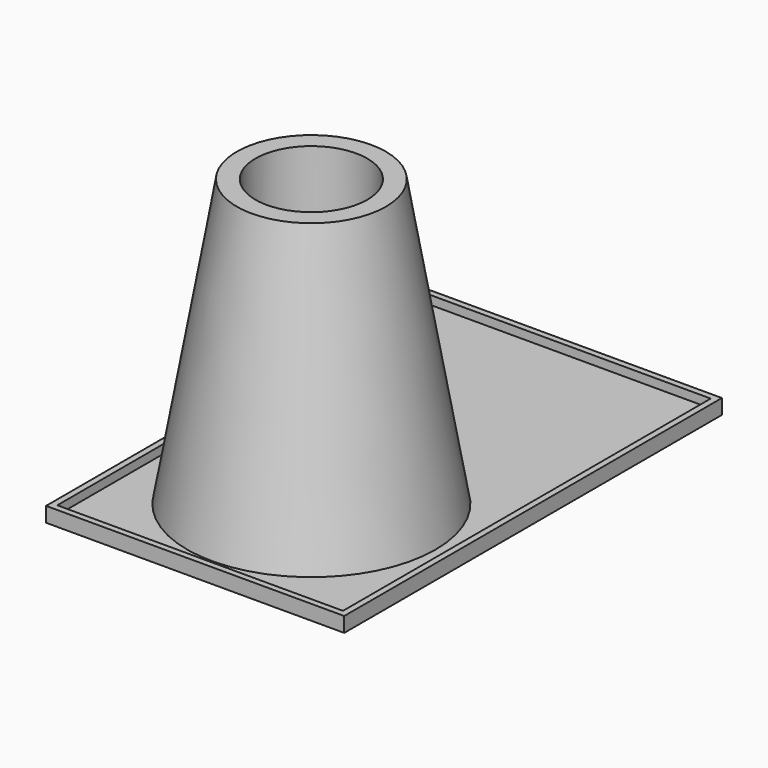
from build123d import *

# Parameters (mm, degrees)
F0_W     = 120
F0_H     = 190
F1_DEPTH = 6
F2_T     = -2.5
F3_R     = 50
F4_DEPTH = 115
F5_SIZE2 = 114.99999
F5_SIZE  = 19.99999
F6_R     = 22.5
F7_DEPTH = 25


# Not quite as in the source:
# - a fillet or chamfer is up to 0.001 mm smaller than in the source, because OpenCascade refuses the exact size


with BuildPart() as f1:
    # F0 (on Top) → F1 (new body)
    with BuildSketch(Plane.XY):
        with Locations((0, 36.5384568274)):
            Rectangle(F0_W, F0_H)
    extrude(amount=F1_DEPTH)

    # F2
    f2_openings = [f1.faces().sort_by_distance(p)[0] for p in [
        (0, 36.538457, 6),
    ]]
    offset(amount=F2_T, openings=f2_openings)

    # F3 (on face) → F4 (join)
    with BuildSketch(Plane.XY.offset(2.5)):
        Circle(F3_R)
    extrude(amount=F4_DEPTH)

    # F5 (size 20 and 115 in the source; OpenCascade refuses exactly that, so slightly less here)
    f5_edges = [f1.edges().sort_by_distance(p)[0] for p in [
        (-50, 0, 117.5),
    ]]
    f5_side = f1.faces().sort_by_distance((0, 0, 117.5))[0]
    chamfer(f5_edges, length=F5_SIZE, length2=F5_SIZE2, reference=f5_side)

    # F6 (on face) → F7 (cut)
    with BuildSketch(Plane.XY.offset(117.5)):
        Circle(F6_R)
    extrude(amount=-F7_DEPTH, mode=Mode.SUBTRACT)


solid = f1.part
